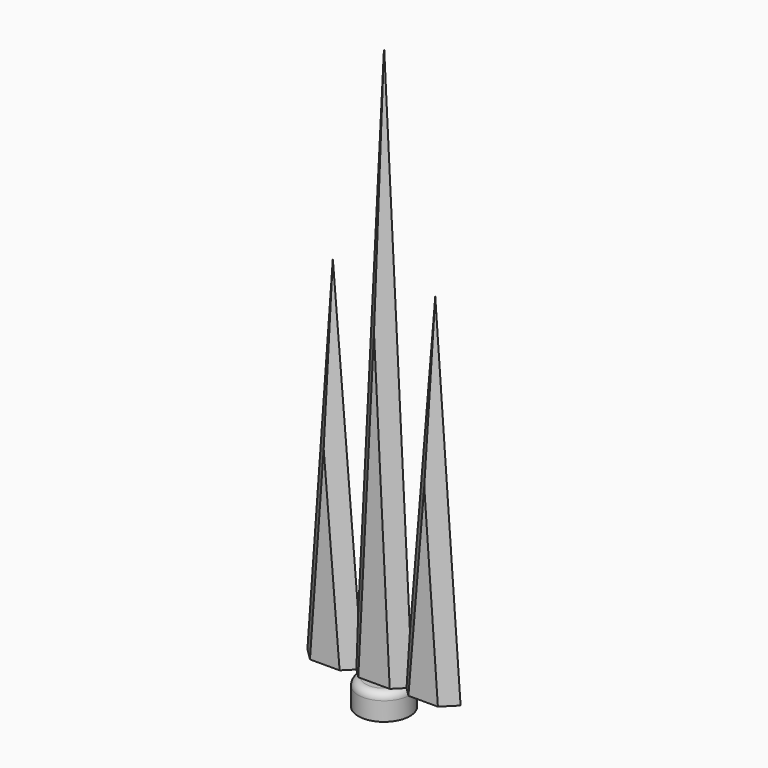
from build123d import *

# Parameters (mm, degrees)
F1_DEPTH     = 3.175
F0_W         = 6.517579814
F0_H         = 6.517579814
F3_R         = 1.8396307345
F4_T1_DEPTH  = 105.2601198415
F4_T3_DEPTH  = 105.2587122864
F4_T8_DEPTH  = 160.6437057027
F4_T13_DEPTH = 160.6437057027
F4_T18_DEPTH = 109.3610790882
F4_T23_DEPTH = 109.3627110349
F4_T28_DEPTH = 109.3610790882
F4_T33_DEPTH = 160.6437057027
F4_T38_DEPTH = 160.6437057027
F4_T43_DEPTH = 109.3627110349
F4_T49_DEPTH = 109.3627110349
F4_T53_DEPTH = 160.6437057027
F4_T60_DEPTH = 160.6437057027
F4_T64_DEPTH = 109.3610790882
F4_T71_DEPTH = 160.6437057027
F4_T75_DEPTH = 109.3610790882
F4_T82_DEPTH = 109.3627110349
F4_T86_DEPTH = 160.6437057027


# Not quite as in the source:
# - a fillet or chamfer that OpenCascade refuses, or shapes differently, is made with other operations: its cross-section is extruded or revolved along the edge and cut away or added


with BuildPart() as f1:
    # F0 (on Front) → F1 (new body, symmetric)
    with BuildSketch(Plane.XZ):
        Polygon((5.8152633182, 17.0447041894), (12.3328431322, 17.0447041894), (25.1026526093, 17.0447041894), (18.7177478708, 105.7437211275), (12.3328431322, 29.3092317879), (5.8152633182, 157.1265012026), (-0.7023164958, 29.3092317879), (-7.1067957186, 105.7437211275), (-13.5112749413, 17.0447041894), (-0.7023164958, 17.0447041894), align=None)
    extrude(amount=F1_DEPTH, both=True)

    # F4: chamfer of 3.175 on 12 edges, made by hand

    # F4_s2 → F4_t1 (cut)
    with BuildSketch(Plane(origin=(8.146753536, 0, 112.828694536), x_dir=(0, 1, 0), z_dir=(-0.0720171377, 0, -0.9974033948))):
        Polygon((0, -14.7037023029), (-3.175, -11.5287023029), (-3.175, -14.7037023029), align=None)
        Polygon((0, -14.7037023029), (3.175, -11.5287023029), (3.175, -14.7037023029), align=None)
    extrude(amount=F4_T1_DEPTH, mode=Mode.SUBTRACT)

    # F4_s4 → F4_t3 (cut)
    with BuildSketch(Plane(origin=(-0.5049778086, 0, 7.0151454149), x_dir=(0, 1, 0), z_dir=(-0.0717981628, 0, 0.9974191816))):
        Polygon((-3.175, -23.0866456679), (0, -26.2616456679), (-3.175, -26.2616456679), align=None)
        Polygon((0, -26.2616456679), (3.175, -23.0866456679), (3.175, -26.2616456679), align=None)
    extrude(amount=F4_T3_DEPTH, mode=Mode.SUBTRACT)


with BuildPart() as f2:
    # F0 (on Front) → F2 (revolve)
    with BuildSketch(Plane.XZ):
        with Locations((2.5564734112, 13.7859142824)):
            Rectangle(F0_W, F0_H)
    revolve(axis=Axis((5.8152633182, 0, 13.7859142824), (0, 0, -1)))

    # F3
    f3_edges = [f2.edges().sort_by_distance(p)[0] for p in [
        (12.332843, 0, 17.044704),
    ]]
    fillet(f3_edges, radius=F3_R)


with BuildPart() as f4_tool6:
    # F4_s7 → F4_t8 (new body)
    with BuildSketch(Plane(origin=(8.4222101757, 0, 165.1692710805), x_dir=(0, 1, 0), z_dir=(-0.0509252238, 0, -0.998702469))):
        Polygon((0, -2.193984407), (-3.175, 0.981015593), (-3.175, -2.193984407), align=None)
    extrude(amount=F4_T8_DEPTH)

    split(bisect_by=Plane(origin=(1.7412915039, 0, 0.1459035751), x_dir=(0, 1, 0), z_dir=(0.9965079584, 0, 0.0834978368)), keep=Keep.TOP)


with BuildPart() as f1_1:
    add(f1.part)

    # F4_t5: cut F4_tool6
    add(f4_tool6.part, mode=Mode.SUBTRACT)


with BuildPart() as f4_tool11:
    # F4_s12 → F4_t13 (new body)
    with BuildSketch(Plane(origin=(-0.2112311518, 0, 4.1424869054), x_dir=(0, 1, 0), z_dir=(-0.0509252238, 0, 0.998702469))):
        Polygon((0, -13.8094200745), (-3.175, -10.6344200745), (-3.175, -13.8094200745), align=None)
    extrude(amount=F4_T13_DEPTH)

    split(bisect_by=Plane(origin=(9.8160197033, 0, -0.8199747425), x_dir=(0, 1, 0), z_dir=(-0.996529161, 0, 0.0832444073)), keep=Keep.TOP)


with BuildPart() as f1_2:
    add(f1_1.part)

    # F4_t10: cut F4_tool11
    add(f4_tool11.part, mode=Mode.SUBTRACT)


with BuildPart() as f4_tool16:
    # F4_s17 → F4_t18 (new body)
    with BuildSketch(Plane(origin=(9.5814265353, 0, 114.7004496316), x_dir=(0, 1, 0), z_dir=(-0.0832444073, 0, -0.996529161))):
        Polygon((0, 9.8502081904), (-3.175, 13.0252081904), (-3.175, 9.8502081904), align=None)
    extrude(amount=F4_T18_DEPTH)

    split(bisect_by=Plane(origin=(13.7915019238, 0, 0.703247808), x_dir=(0, 1, 0), z_dir=(0.998702469, 0, 0.0509252238)), keep=Keep.TOP)


with BuildPart() as f1_3:
    add(f1_2.part)

    # F4_t15: cut F4_tool16
    add(f4_tool16.part, mode=Mode.SUBTRACT)


with BuildPart() as f4_tool21:
    # F4_s22 → F4_t23 (new body)
    with BuildSketch(Plane(origin=(-0.39830507, 0, 4.7535862896), x_dir=(0, 1, 0), z_dir=(-0.0834978368, 0, 0.9965079584))):
        Polygon((0, -1.7473934745), (-3.175, 1.4276065255), (-3.175, -1.7473934745), align=None)
    extrude(amount=F4_T23_DEPTH)

    split(bisect_by=Plane(origin=(-2.1911376442, 0, 0.111729147), x_dir=(0, 1, 0), z_dir=(-0.998702469, 0, 0.0509252238)), keep=Keep.TOP)


with BuildPart() as f1_4:
    add(f1_3.part)

    # F4_t20: cut F4_tool21
    add(f4_tool21.part, mode=Mode.SUBTRACT)


with BuildPart() as f4_tool26:
    # F4_s27 → F4_t28 (new body)
    with BuildSketch(Plane(origin=(9.5814265353, 0, 114.7004496316), x_dir=(0, 1, 0), z_dir=(-0.0832444073, 0, -0.996529161))):
        Polygon((0, 9.8502081904), (3.175, 13.0252081904), (3.175, 9.8502081904), align=None)
    extrude(amount=F4_T28_DEPTH)

    split(bisect_by=Plane(origin=(13.7915019238, 0, 0.703247808), x_dir=(0, 1, 0), z_dir=(0.998702469, 0, 0.0509252238)), keep=Keep.TOP)


with BuildPart() as f1_5:
    add(f1_4.part)

    # F4_t25: cut F4_tool26
    add(f4_tool26.part, mode=Mode.SUBTRACT)


with BuildPart() as f4_tool31:
    # F4_s32 → F4_t33 (new body)
    with BuildSketch(Plane(origin=(-0.2112311518, 0, 4.1424869054), x_dir=(0, 1, 0), z_dir=(-0.0509252238, 0, 0.998702469))):
        Polygon((0, -13.8094200745), (3.175, -10.6344200745), (3.175, -13.8094200745), align=None)
    extrude(amount=F4_T33_DEPTH)

    split(bisect_by=Plane(origin=(9.8160197033, 0, -0.8199747425), x_dir=(0, 1, 0), z_dir=(-0.996529161, 0, 0.0832444073)), keep=Keep.TOP)


with BuildPart() as f1_6:
    add(f1_5.part)

    # F4_t30: cut F4_tool31
    add(f4_tool31.part, mode=Mode.SUBTRACT)


with BuildPart() as f4_tool36:
    # F4_s37 → F4_t38 (new body)
    with BuildSketch(Plane(origin=(8.4222101757, 0, 165.1692710805), x_dir=(0, 1, 0), z_dir=(-0.0509252238, 0, -0.998702469))):
        Polygon((0, -2.193984407), (3.175, 0.981015593), (3.175, -2.193984407), align=None)
    extrude(amount=F4_T38_DEPTH)

    split(bisect_by=Plane(origin=(1.7412915039, 0, 0.1459035751), x_dir=(0, 1, 0), z_dir=(0.9965079584, 0, 0.0834978368)), keep=Keep.TOP)


with BuildPart() as f1_7:
    add(f1_6.part)

    # F4_t35: cut F4_tool36
    add(f4_tool36.part, mode=Mode.SUBTRACT)


with BuildPart() as f4_tool41:
    # F4_s42 → F4_t43 (new body)
    with BuildSketch(Plane(origin=(-0.39830507, 0, 4.7535862896), x_dir=(0, 1, 0), z_dir=(-0.0834978368, 0, 0.9965079584))):
        Polygon((0, -1.7473934745), (3.175, 1.4276065255), (3.175, -1.7473934745), align=None)
    extrude(amount=F4_T43_DEPTH)

    split(bisect_by=Plane(origin=(-2.1911376442, 0, 0.111729147), x_dir=(0, 1, 0), z_dir=(-0.998702469, 0, 0.0509252238)), keep=Keep.TOP)


with BuildPart() as f1_8:
    add(f1_7.part)

    # F4_t40: cut F4_tool41
    add(f4_tool41.part, mode=Mode.SUBTRACT)


with BuildPart() as f4_tool47:
    # F4_s48 → F4_t49 (new body)
    with BuildSketch(Plane(origin=(-0.39830507, 0, 4.7535862896), x_dir=(0, 1, 0), z_dir=(-0.0834978368, 0, 0.9965079584))):
        Polygon((0, -1.7473934745), (-3.175, 1.4276065255), (-3.175, -1.7473934745), align=None)
    extrude(amount=F4_T49_DEPTH)

    split(bisect_by=Plane(origin=(-2.1911376442, 0, 0.111729147), x_dir=(0, 1, 0), z_dir=(0.998702469, 0, -0.0509252238)), keep=Keep.TOP)


with BuildPart() as f4_tool51:
    # F4_s52 → F4_t53 (new body)
    with BuildSketch(Plane(origin=(8.4222101757, 0, 165.1692710805), x_dir=(0, 1, 0), z_dir=(-0.0509252238, 0, -0.998702469))):
        Polygon((0, -2.193984407), (-3.175, 0.981015593), (-3.175, -2.193984407), align=None)
    extrude(amount=F4_T53_DEPTH)

    split(bisect_by=Plane(origin=(1.7412915039, 0, 0.1459035751), x_dir=(0, 1, 0), z_dir=(-0.9965079584, 0, -0.0834978368)), keep=Keep.TOP)


with BuildPart() as f4_tool47_1:
    add(f4_tool47.part)

    # F4_t55: intersect F4_tool51
    add(f4_tool51.part, mode=Mode.INTERSECT)


with BuildPart() as f1_9:
    add(f1_8.part)

    # F4_t45: cut F4_tool47
    add(f4_tool47_1.part, mode=Mode.SUBTRACT)


with BuildPart() as f4_tool58:
    # F4_s59 → F4_t60 (new body)
    with BuildSketch(Plane(origin=(-0.2112311518, 0, 4.1424869054), x_dir=(0, 1, 0), z_dir=(-0.0509252238, 0, 0.998702469))):
        Polygon((0, -13.8094200745), (-3.175, -10.6344200745), (-3.175, -13.8094200745), align=None)
    extrude(amount=F4_T60_DEPTH)

    split(bisect_by=Plane(origin=(9.8160197033, 0, -0.8199747425), x_dir=(0, 1, 0), z_dir=(0.996529161, 0, -0.0832444073)), keep=Keep.TOP)


with BuildPart() as f4_tool62:
    # F4_s63 → F4_t64 (new body)
    with BuildSketch(Plane(origin=(9.5814265353, 0, 114.7004496316), x_dir=(0, 1, 0), z_dir=(-0.0832444073, 0, -0.996529161))):
        Polygon((0, 9.8502081904), (-3.175, 13.0252081904), (-3.175, 9.8502081904), align=None)
    extrude(amount=F4_T64_DEPTH)

    split(bisect_by=Plane(origin=(13.7915019238, 0, 0.703247808), x_dir=(0, 1, 0), z_dir=(-0.998702469, 0, -0.0509252238)), keep=Keep.TOP)


with BuildPart() as f4_tool58_1:
    add(f4_tool58.part)

    # F4_t66: intersect F4_tool62
    add(f4_tool62.part, mode=Mode.INTERSECT)


with BuildPart() as f1_10:
    add(f1_9.part)

    # F4_t56: cut F4_tool58
    add(f4_tool58_1.part, mode=Mode.SUBTRACT)


with BuildPart() as f4_tool69:
    # F4_s70 → F4_t71 (new body)
    with BuildSketch(Plane(origin=(-0.2112311518, 0, 4.1424869054), x_dir=(0, 1, 0), z_dir=(-0.0509252238, 0, 0.998702469))):
        Polygon((0, -13.8094200745), (3.175, -10.6344200745), (3.175, -13.8094200745), align=None)
    extrude(amount=F4_T71_DEPTH)

    split(bisect_by=Plane(origin=(9.8160197033, 0, -0.8199747425), x_dir=(0, 1, 0), z_dir=(0.996529161, 0, -0.0832444073)), keep=Keep.TOP)


with BuildPart() as f4_tool73:
    # F4_s74 → F4_t75 (new body)
    with BuildSketch(Plane(origin=(9.5814265353, 0, 114.7004496316), x_dir=(0, 1, 0), z_dir=(-0.0832444073, 0, -0.996529161))):
        Polygon((0, 9.8502081904), (3.175, 13.0252081904), (3.175, 9.8502081904), align=None)
    extrude(amount=F4_T75_DEPTH)

    split(bisect_by=Plane(origin=(13.7915019238, 0, 0.703247808), x_dir=(0, 1, 0), z_dir=(-0.998702469, 0, -0.0509252238)), keep=Keep.TOP)


with BuildPart() as f4_tool69_1:
    add(f4_tool69.part)

    # F4_t77: intersect F4_tool73
    add(f4_tool73.part, mode=Mode.INTERSECT)


with BuildPart() as f1_11:
    add(f1_10.part)

    # F4_t67: cut F4_tool69
    add(f4_tool69_1.part, mode=Mode.SUBTRACT)


with BuildPart() as f4_tool80:
    # F4_s81 → F4_t82 (new body)
    with BuildSketch(Plane(origin=(-0.39830507, 0, 4.7535862896), x_dir=(0, 1, 0), z_dir=(-0.0834978368, 0, 0.9965079584))):
        Polygon((0, -1.7473934745), (3.175, 1.4276065255), (3.175, -1.7473934745), align=None)
    extrude(amount=F4_T82_DEPTH)

    split(bisect_by=Plane(origin=(-2.1911376442, 0, 0.111729147), x_dir=(0, 1, 0), z_dir=(0.998702469, 0, -0.0509252238)), keep=Keep.TOP)


with BuildPart() as f4_tool84:
    # F4_s85 → F4_t86 (new body)
    with BuildSketch(Plane(origin=(8.4222101757, 0, 165.1692710805), x_dir=(0, 1, 0), z_dir=(-0.0509252238, 0, -0.998702469))):
        Polygon((0, -2.193984407), (3.175, 0.981015593), (3.175, -2.193984407), align=None)
    extrude(amount=F4_T86_DEPTH)

    split(bisect_by=Plane(origin=(1.7412915039, 0, 0.1459035751), x_dir=(0, 1, 0), z_dir=(-0.9965079584, 0, -0.0834978368)), keep=Keep.TOP)


with BuildPart() as f4_tool80_1:
    add(f4_tool80.part)

    # F4_t88: intersect F4_tool84
    add(f4_tool84.part, mode=Mode.INTERSECT)


with BuildPart() as f1_12:
    add(f1_11.part)

    # F4_t78: cut F4_tool80
    add(f4_tool80_1.part, mode=Mode.SUBTRACT)


solid = Compound([f2.part, f1_12.part])
